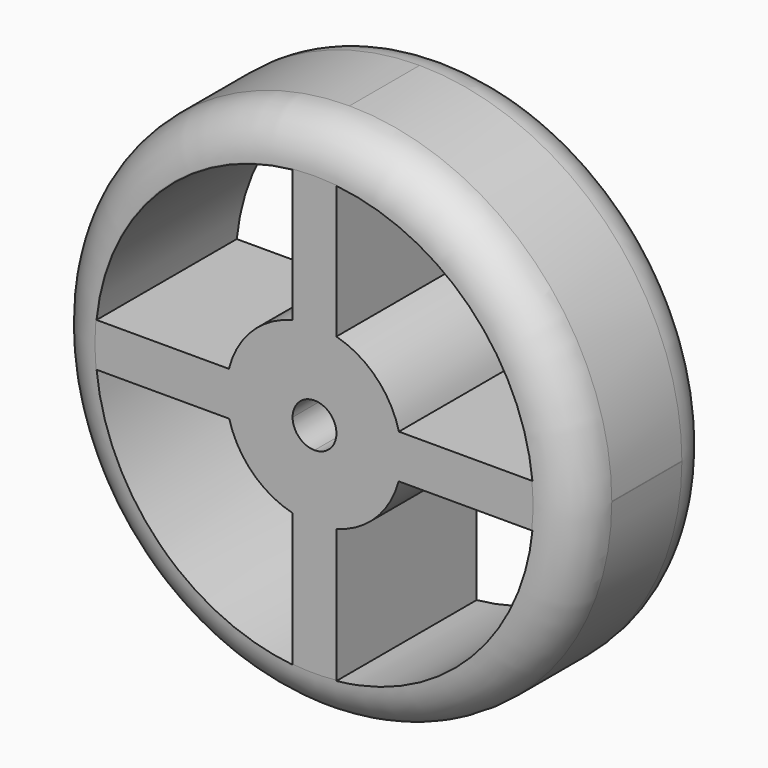
from build123d import *

# Parameters (mm, degrees)
F1_DEPTH = 20


# Not quite as in the source:
# - a fillet or chamfer that OpenCascade refuses, or shapes differently, is made with other operations: its cross-section is extruded or revolved along the edge and cut away or added


with BuildPart() as f1:
    # F0 (on Front) → F1 (new body)
    with BuildSketch(Plane.XZ):
        with BuildLine():
            ThreePointArc((29.999922187, -0.0683284437), (29.9999805467, -0.034164244), (30, 0))
            ThreePointArc((30, 0), (21.2373474192, 21.189031941), (0.0683283603, 29.9999221872))
            Line((0.0683283603, 29.9999221872), (0.0683283603, 2.4316715563))
            ThreePointArc((0.0683283603, 2.4316715563), (1.8360953132, 1.6994385093), (2.5683283603, -0.0683284437))
            Line((2.5683283603, -0.0683284437), (29.999922187, -0.0683284437))
        make_face()
        with BuildLine():
            Line((24.9431081335, 2.4307376289), (9.7000780708, 2.4307376289))
            ThreePointArc((9.7000780708, 2.4307376289), (7.1211298187, 7.0206488379), (2.5683283603, 9.664558419))
            Line((2.5683283603, 9.664558419), (2.5683283603, 24.806357484))
            ThreePointArc((2.5683283603, 24.806357484), (17.7463297429, 17.6090092268), (24.9431081335, 2.4307376289))
        make_face(mode=Mode.SUBTRACT)
        with BuildLine():
            Line((0.0683283603, 2.4316715563), (0.0683283603, 29.9999221872))
            ThreePointArc((0.0683283603, 29.9999221872), (-21.2132034651, 21.2132034061), (-29.999922187, -0.0683284437))
            Line((-29.999922187, -0.0683284437), (-2.4316716397, -0.0683284437))
            ThreePointArc((-2.4316716397, -0.0683284437), (-1.7234334683, 1.675113425), (0, 2.4307376289))
            ThreePointArc((0, 2.4307376289), (0.034160989, 2.4314380635), (0.0683283603, 2.4316715563))
        make_face()
        with BuildLine():
            ThreePointArc((-24.8064514129, 2.4307376289), (-17.6096730223, 17.6090092268), (-2.4316716397, 24.806357484))
            Line((-2.4316716397, 24.806357484), (-2.4316716397, 9.6998439697))
            ThreePointArc((-2.4316716397, 9.6998439697), (-7.0714082408, 7.0707273665), (-9.7000780708, 2.4307376289))
            Line((-9.7000780708, 2.4307376289), (-24.8064514129, 2.4307376289))
        make_face(mode=Mode.SUBTRACT)
        with BuildLine():
            ThreePointArc((0.0683283603, -29.9999221872), (21.2132034061, -21.2132034651), (29.999922187, -0.0683284437))
            Line((29.999922187, -0.0683284437), (2.5683283603, -0.0683284437))
            ThreePointArc((2.5683283603, -0.0683284437), (1.8360953132, -1.8360953967), (0.0683283603, -2.5683284437))
            Line((0.0683283603, -2.5683284437), (0.0683283603, -29.9999221872))
        make_face()
        with BuildLine():
            ThreePointArc((24.9430142879, -2.5683284437), (17.7459978899, -17.7459979734), (2.5683283603, -24.9430143714))
            Line((2.5683283603, -24.9430143714), (2.5683283603, -9.664558419))
            ThreePointArc((2.5683283603, -9.664558419), (7.0710677813, -7.0710678424), (9.6645583968, -2.5683284437))
            Line((9.6645583968, -2.5683284437), (24.9430142879, -2.5683284437))
        make_face(mode=Mode.SUBTRACT)
        with BuildLine():
            Line((-2.4316716397, -0.0683284437), (-29.999922187, -0.0683284437))
            ThreePointArc((-29.999922187, -0.0683284437), (-21.1648329371, -21.2614638899), (0.0683283603, -29.9999221872))
            Line((0.0683283603, -29.9999221872), (0.0683283603, -2.5683284437))
            ThreePointArc((0.0683283603, -2.5683284437), (-1.6994385927, -1.8360953967), (-2.4316716397, -0.0683284437))
        make_face()
        with BuildLine():
            ThreePointArc((-2.4316716397, -24.9430143714), (-17.6093411694, -17.7459979734), (-24.8063575674, -2.5683284437))
            Line((-24.8063575674, -2.5683284437), (-9.6645583968, -2.5683284437))
            ThreePointArc((-9.6645583968, -2.5683284437), (-7.0209916464, -7.1207918311), (-2.4316716397, -9.6998439697))
            Line((-2.4316716397, -9.6998439697), (-2.4316716397, -24.9430143714))
        make_face(mode=Mode.SUBTRACT)
    extrude(amount=F1_DEPTH)

    # F2: fillet of radius 5 on 1 edges, made by hand

    # F2_s1 → F2_t2 (revolve, cut)
    with BuildSketch(Plane(origin=(0, 0, 0), x_dir=(0, 1, 0), z_dir=(-0.0022776148, 0, 0.9999974062))):
        with BuildLine():
            ThreePointArc((-15, 30), (-18.5355339059, 28.5355339059), (-20, 25))
            Line((-20, 25), (-20, 30))
            Line((-20, 30), (-15, 30))
        make_face()
    revolve(axis=Axis((0, -20, 0), (0, -1, 0)), mode=Mode.SUBTRACT)

    # F3: fillet of radius 5 on 1 edges, made by hand

    # F3_s1 → F3_t2 (revolve, cut)
    with BuildSketch(Plane(origin=(0, 0, 0), x_dir=(0, 1, 0), z_dir=(-0.0022776148, 0, 0.9999974062))):
        with BuildLine():
            ThreePointArc((0, 25), (-1.4644660941, 28.5355339059), (-5, 30))
            Line((-5, 30), (0, 30))
            Line((0, 30), (0, 25))
        make_face()
    revolve(axis=Axis((0, 0, 0), (0, -1, 0)), mode=Mode.SUBTRACT)


solid = f1.part
